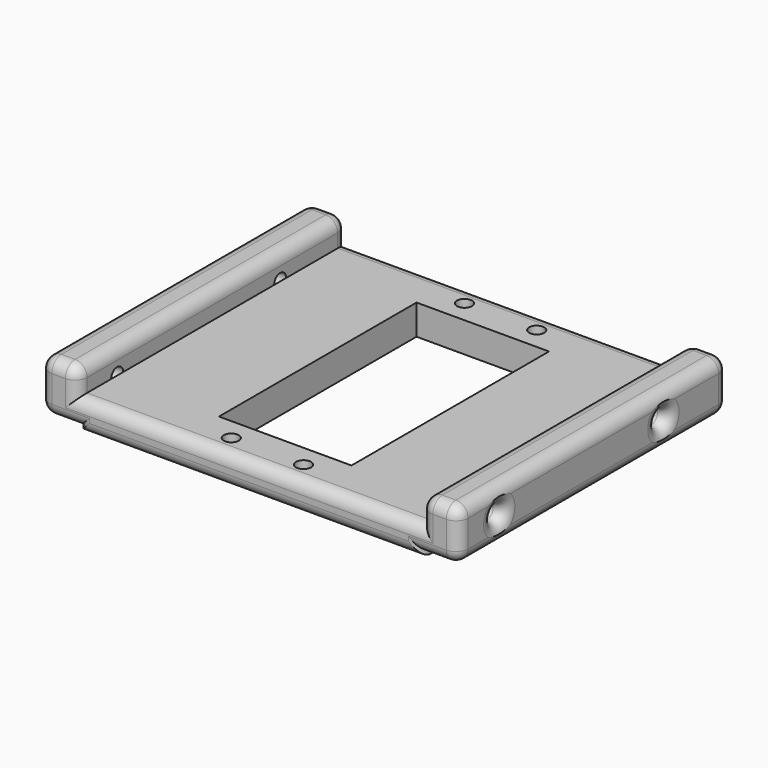
from build123d import *

# Parameters (mm, degrees)
F0_W           = 57
F0_H           = 56
F0_W_2         = 22
F0_H_2         = 41
F1_DEPTH       = 5
F3_W           = 56
F3_H           = 8.5
F4_DEPTH       = 6.25
F6_W           = 56
F6_H           = 8.5
F7_DEPTH       = 6.25
F8_D           = 2.5
F9_D           = 2.5
F9_DEPTH       = 6.251
F10_D          = 2.5
F10_DEPTH      = 6.251
F11_T1_DEPTH   = 2.25
F11_T3_DEPTH   = 52
F11_T5_DEPTH   = 4.5
F11_T7_DEPTH   = 5.75
F11_T9_DEPTH   = 67
F11_T11_DEPTH  = 4.25
F11_T13_DEPTH  = 2.25
F11_T15_DEPTH  = 57
F11_T17_DEPTH  = 2.25
F11_T19_DEPTH  = 4.25
F11_S23_W      = 2
F11_S23_H      = 2
F11_T24_DEPTH  = 2
F11_S29_W      = 2
F11_S29_H      = 2
F11_T30_DEPTH  = 2
F11_S35_W      = 2
F11_S35_H      = 2
F11_T36_DEPTH  = 2
F11_S41_W      = 2
F11_S41_H      = 2
F11_T42_DEPTH  = 2
F11_S47_W      = 2
F11_S47_H      = 2
F11_T48_DEPTH  = 2
F11_S53_W      = 2
F11_S53_H      = 2
F11_T54_DEPTH  = 2
F11_S59_W      = 2
F11_S59_H      = 2
F11_T60_DEPTH  = 2
F11_S65_W      = 2
F11_S65_H      = 2
F11_T66_DEPTH  = 2
F11_S71_W      = 2
F11_S71_H      = 2
F11_T72_DEPTH  = 2
F11_S77_W      = 2
F11_S77_H      = 2
F11_T78_DEPTH  = 2
F11_S83_W      = 2
F11_S83_H      = 2
F11_T84_DEPTH  = 2
F11_S89_W      = 2
F11_S89_H      = 2
F11_T90_DEPTH  = 2
F11_T105_DEPTH = 10.75
F11_T109_DEPTH = 9.25
F11_T116_DEPTH = 10.75
F11_T120_DEPTH = 9.25
F11_T127_DEPTH = 7.25
F11_T131_DEPTH = 62
F11_T138_DEPTH = 62
F11_T142_DEPTH = 7.25
F11_T149_DEPTH = 10.75
F11_T153_DEPTH = 9.25
F11_T160_DEPTH = 10.75
F11_T164_DEPTH = 9.25
F11_T171_DEPTH = 62
F11_T175_DEPTH = 7.25
F11_T182_DEPTH = 7.25
F11_T186_DEPTH = 62


# Not quite as in the source:
# - a fillet or chamfer that OpenCascade refuses, or shapes differently, is made with other operations: its cross-section is extruded or revolved along the edge and cut away or added


with BuildPart() as f1:
    # F0 (on Top) → F1 (new body)
    with BuildSketch(Plane.XY):
        Rectangle(F0_W, F0_H)
        Rectangle(F0_W_2, F0_H_2, mode=Mode.SUBTRACT)
    extrude(amount=-F1_DEPTH)

    # F3 (on offset) → F4 (join)
    with BuildSketch(Plane(origin=(-28.5, 0, 0), x_dir=(0, -1, 0), z_dir=(-1, 0, 0))):
        Rectangle(F3_W, F3_H)
    extrude(amount=F4_DEPTH)

    # F6 (on offset) → F7 (join)
    with BuildSketch(Plane.YZ.offset(28.5)):
        Rectangle(F6_W, F6_H)
    extrude(amount=F7_DEPTH)

    # F8 (through all)
    with Locations(Plane.XY):
        with Locations((6, 24.2), (-6, 24.2), (-6, -24.2), (6, -24.2)):
            Hole(F8_D / 2)

    # F9 (through all, one way)
    with BuildSketch(Plane(origin=(-28.5, 0, 0), x_dir=(0, -1, 0), z_dir=(1, 0, 0))):
        with Locations((-14.0771195292, 0), (19.7577979416, 0)):
            Circle(F9_D / 2)
    extrude(amount=-F9_DEPTH, mode=Mode.SUBTRACT)

    # F10 (through all, one way)
    with BuildSketch(Plane(origin=(28.5, 0, 0), x_dir=(0, 1, 0), z_dir=(-1, 0, 0))):
        with Locations((-19.5172671229, 0), (14.5558202639, 0)):
            Circle(F10_D / 2)
    extrude(amount=-F10_DEPTH, mode=Mode.SUBTRACT)

    # F11: fillet of radius 2 on 34 edges, made by hand

    # F11_s2 → F11_t1 (cut)
    with BuildSketch(Plane.YZ.offset(30.5)):
        with BuildLine():
            ThreePointArc((26, 4.25), (27.4142135624, 3.6642135624), (28, 2.25))
            Line((28, 2.25), (28, 4.25))
            Line((28, 4.25), (26, 4.25))
        make_face()
        with BuildLine():
            ThreePointArc((-28, 2.25), (-27.4142135624, 3.6642135624), (-26, 4.25))
            Line((-26, 4.25), (-28, 4.25))
            Line((-28, 4.25), (-28, 2.25))
        make_face()
    extrude(amount=F11_T1_DEPTH, mode=Mode.SUBTRACT)

    # F11_s4 → F11_t3 (cut)
    with BuildSketch(Plane.XZ.offset(-26)):
        with BuildLine():
            ThreePointArc((30.5, 4.25), (29.0857864376, 3.6642135624), (28.5, 2.25))
            Line((28.5, 2.25), (28.5, 4.25))
            Line((28.5, 4.25), (30.5, 4.25))
        make_face()
        with BuildLine():
            ThreePointArc((34.75, 2.25), (34.1642135624, 3.6642135624), (32.75, 4.25))
            Line((32.75, 4.25), (34.75, 4.25))
            Line((34.75, 4.25), (34.75, 2.25))
        make_face()
        with BuildLine():
            ThreePointArc((32.75, -4.25), (34.1642135624, -3.6642135624), (34.75, -2.25))
            Line((34.75, -2.25), (34.75, -4.25))
            Line((34.75, -4.25), (32.75, -4.25))
        make_face()
        with BuildLine():
            ThreePointArc((-28.5, 2.25), (-29.0857864376, 3.6642135624), (-30.5, 4.25))
            Line((-30.5, 4.25), (-28.5, 4.25))
            Line((-28.5, 4.25), (-28.5, 2.25))
        make_face()
        with BuildLine():
            ThreePointArc((-32.75, 4.25), (-34.1642135624, 3.6642135624), (-34.75, 2.25))
            Line((-34.75, 2.25), (-34.75, 4.25))
            Line((-34.75, 4.25), (-32.75, 4.25))
        make_face()
        with BuildLine():
            ThreePointArc((-34.75, -2.25), (-34.1642135624, -3.6642135624), (-32.75, -4.25))
            Line((-32.75, -4.25), (-34.75, -4.25))
            Line((-34.75, -4.25), (-34.75, -2.25))
        make_face()
    extrude(amount=F11_T3_DEPTH, mode=Mode.SUBTRACT)

    # F11_s6 → F11_t5 (cut)
    with BuildSketch(Plane.XY.offset(-2.25)):
        with BuildLine():
            ThreePointArc((32.75, -28), (34.1642135624, -27.4142135624), (34.75, -26))
            Line((34.75, -26), (34.75, -28))
            Line((34.75, -28), (32.75, -28))
        make_face()
        with BuildLine():
            ThreePointArc((34.75, 26), (34.1642135624, 27.4142135624), (32.75, 28))
            Line((32.75, 28), (34.75, 28))
            Line((34.75, 28), (34.75, 26))
        make_face()
        with BuildLine():
            ThreePointArc((-32.75, -28), (-34.1642135624, -27.4142135624), (-34.75, -26))
            Line((-34.75, -26), (-34.75, -28))
            Line((-34.75, -28), (-32.75, -28))
        make_face()
        with BuildLine():
            ThreePointArc((-34.75, 26), (-34.1642135624, 27.4142135624), (-32.75, 28))
            Line((-32.75, 28), (-34.75, 28))
            Line((-34.75, 28), (-34.75, 26))
        make_face()
    extrude(amount=F11_T5_DEPTH, mode=Mode.SUBTRACT)

    # F11_s8 → F11_t7 (cut)
    with BuildSketch(Plane.XY.offset(-10)):
        with BuildLine():
            ThreePointArc((-26.5, -28), (-27.9142135624, -27.4142135624), (-28.5, -26))
            Line((-28.5, -26), (-28.5, -28))
            Line((-28.5, -28), (-26.5, -28))
        make_face()
        with BuildLine():
            ThreePointArc((26.5, -28), (27.9142135624, -27.4142135624), (28.5, -26))
            Line((28.5, -26), (28.5, -28))
            Line((28.5, -28), (26.5, -28))
        make_face()
        with BuildLine():
            ThreePointArc((28.5, 26), (27.9142135624, 27.4142135624), (26.5, 28))
            Line((26.5, 28), (28.5, 28))
            Line((28.5, 28), (28.5, 26))
        make_face()
        with BuildLine():
            ThreePointArc((-28.5, 26), (-27.9142135624, 27.4142135624), (-26.5, 28))
            Line((-26.5, 28), (-28.5, 28))
            Line((-28.5, 28), (-28.5, 26))
        make_face()
    extrude(amount=F11_T7_DEPTH, mode=Mode.SUBTRACT)

    # F11_s10 → F11_t9 (cut)
    with BuildSketch(Plane.YZ.offset(-33.5)):
        with BuildLine():
            ThreePointArc((-28, -3), (-27.4142135624, -4.4142135624), (-26, -5))
            Line((-26, -5), (-28, -5))
            Line((-28, -5), (-28, -3))
        make_face()
        with BuildLine():
            ThreePointArc((26, -5), (27.4142135624, -4.4142135624), (28, -3))
            Line((28, -3), (28, -5))
            Line((28, -5), (26, -5))
        make_face()
    extrude(amount=F11_T9_DEPTH, mode=Mode.SUBTRACT)

    # F11_s12 → F11_t11 (cut)
    with BuildSketch(Plane.YZ.offset(28.5)):
        with BuildLine():
            ThreePointArc((-28, -2.25), (-27.4142135624, -3.6642135624), (-26, -4.25))
            Line((-26, -4.25), (-28, -4.25))
            Line((-28, -4.25), (-28, -2.25))
        make_face()
        with BuildLine():
            ThreePointArc((26, -4.25), (27.4142135624, -3.6642135624), (28, -2.25))
            Line((28, -2.25), (28, -4.25))
            Line((28, -4.25), (26, -4.25))
        make_face()
    extrude(amount=F11_T11_DEPTH, mode=Mode.SUBTRACT)

    # F11_s14 → F11_t13 (cut)
    with BuildSketch(Plane.XY):
        with BuildLine():
            ThreePointArc((30.5, -28), (29.0857864376, -27.4142135624), (28.5, -26))
            Line((28.5, -26), (28.5, -28))
            Line((28.5, -28), (30.5, -28))
        make_face()
        with BuildLine():
            ThreePointArc((-30.5, -28), (-29.0857864376, -27.4142135624), (-28.5, -26))
            Line((-28.5, -26), (-28.5, -28))
            Line((-28.5, -28), (-30.5, -28))
        make_face()
        with BuildLine():
            ThreePointArc((-28.5, 26), (-29.0857864376, 27.4142135624), (-30.5, 28))
            Line((-30.5, 28), (-28.5, 28))
            Line((-28.5, 28), (-28.5, 26))
        make_face()
        with BuildLine():
            ThreePointArc((28.5, 26), (29.0857864376, 27.4142135624), (30.5, 28))
            Line((30.5, 28), (28.5, 28))
            Line((28.5, 28), (28.5, 26))
        make_face()
    extrude(amount=F11_T13_DEPTH, mode=Mode.SUBTRACT)

    # F11_s16 → F11_t15 (cut)
    with BuildSketch(Plane.YZ.offset(-28.5)):
        with BuildLine():
            ThreePointArc((-28, -2), (-27.4142135624, -0.5857864376), (-26, 0))
            Line((-26, 0), (-28, 0))
            Line((-28, 0), (-28, -2))
        make_face()
        with BuildLine():
            ThreePointArc((26, 0), (27.4142135624, -0.5857864376), (28, -2))
            Line((28, -2), (28, 0))
            Line((28, 0), (26, 0))
        make_face()
    extrude(amount=F11_T15_DEPTH, mode=Mode.SUBTRACT)

    # F11_s18 → F11_t17 (cut)
    with BuildSketch(Plane.YZ.offset(-32.75)):
        with BuildLine():
            ThreePointArc((-28, 2.25), (-27.4142135624, 3.6642135624), (-26, 4.25))
            Line((-26, 4.25), (-28, 4.25))
            Line((-28, 4.25), (-28, 2.25))
        make_face()
        with BuildLine():
            ThreePointArc((26, 4.25), (27.4142135624, 3.6642135624), (28, 2.25))
            Line((28, 2.25), (28, 4.25))
            Line((28, 4.25), (26, 4.25))
        make_face()
    extrude(amount=F11_T17_DEPTH, mode=Mode.SUBTRACT)

    # F11_s20 → F11_t19 (cut)
    with BuildSketch(Plane.YZ.offset(-32.75)):
        with BuildLine():
            ThreePointArc((-28, -2.25), (-27.4142135624, -3.6642135624), (-26, -4.25))
            Line((-26, -4.25), (-28, -4.25))
            Line((-28, -4.25), (-28, -2.25))
        make_face()
        with BuildLine():
            ThreePointArc((26, -4.25), (27.4142135624, -3.6642135624), (28, -2.25))
            Line((28, -2.25), (28, -4.25))
            Line((28, -4.25), (26, -4.25))
        make_face()
    extrude(amount=F11_T19_DEPTH, mode=Mode.SUBTRACT)


with BuildPart() as f11_tool22:
    # F11_s23 → F11_t24 (new body)
    with BuildSketch(Plane.XZ.offset(-26)):
        with Locations((29.5, 3.25)):
            Rectangle(F11_S23_W, F11_S23_H)
    extrude(amount=-F11_T24_DEPTH)

    # F11_s25 → F11_t26 (revolve, cut)
    with BuildSketch(Plane(origin=(30.5, 26, 2.25), x_dir=(0.7071067812, 0, -0.7071067812), z_dir=(0.7071067812, 0, 0.7071067812))):
        with BuildLine():
            ThreePointArc((0, -2), (2, 0), (0, 2))
            Line((0, 2), (0, -2))
        make_face()
    revolve(axis=Axis((30.5, 26, 2.25), (0, 1, 0)), mode=Mode.SUBTRACT)


with BuildPart() as f1_1:
    add(f1.part)

    # F11_t21: cut F11_tool22
    add(f11_tool22.part, mode=Mode.SUBTRACT)


with BuildPart() as f11_tool28:
    # F11_s29 → F11_t30 (new body)
    with BuildSketch(Plane.YZ.offset(32.75)):
        with Locations((27, 3.25)):
            Rectangle(F11_S29_W, F11_S29_H)
    extrude(amount=F11_T30_DEPTH)

    # F11_s31 → F11_t32 (revolve, cut)
    with BuildSketch(Plane(origin=(32.75, 26, 2.25), x_dir=(0, -0.7071067812, -0.7071067812), z_dir=(0, -0.7071067812, 0.7071067812))):
        with BuildLine():
            ThreePointArc((0, -2), (2, 0), (0, 2))
            Line((0, 2), (0, -2))
        make_face()
    revolve(axis=Axis((32.75, 26, 2.25), (1, 0, 0)), mode=Mode.SUBTRACT)


with BuildPart() as f1_2:
    add(f1_1.part)

    # F11_t27: cut F11_tool28
    add(f11_tool28.part, mode=Mode.SUBTRACT)


with BuildPart() as f11_tool34:
    # F11_s35 → F11_t36 (new body)
    with BuildSketch(Plane.XZ.offset(26)):
        with Locations((29.5, 3.25)):
            Rectangle(F11_S35_W, F11_S35_H)
    extrude(amount=F11_T36_DEPTH)

    # F11_s37 → F11_t38 (revolve, cut)
    with BuildSketch(Plane(origin=(30.5, -26, 2.25), x_dir=(0.7071067812, 0, -0.7071067812), z_dir=(-0.7071067812, 0, -0.7071067812))):
        with BuildLine():
            ThreePointArc((0, -2), (2, 0), (0, 2))
            Line((0, 2), (0, -2))
        make_face()
    revolve(axis=Axis((30.5, -26, 2.25), (0, -1, 0)), mode=Mode.SUBTRACT)


with BuildPart() as f1_3:
    add(f1_2.part)

    # F11_t33: cut F11_tool34
    add(f11_tool34.part, mode=Mode.SUBTRACT)


with BuildPart() as f11_tool40:
    # F11_s41 → F11_t42 (new body)
    with BuildSketch(Plane.XZ.offset(26)):
        with Locations((33.75, 3.25)):
            Rectangle(F11_S41_W, F11_S41_H)
    extrude(amount=F11_T42_DEPTH)

    # F11_s43 → F11_t44 (revolve, cut)
    with BuildSketch(Plane(origin=(32.75, -26, 2.25), x_dir=(-0.7071067812, 0, -0.7071067812), z_dir=(-0.7071067812, 0, 0.7071067812))):
        with BuildLine():
            ThreePointArc((0, -2), (2, 0), (0, 2))
            Line((0, 2), (0, -2))
        make_face()
    revolve(axis=Axis((32.75, -26, 2.25), (0, -1, 0)), mode=Mode.SUBTRACT)


with BuildPart() as f1_4:
    add(f1_3.part)

    # F11_t39: cut F11_tool40
    add(f11_tool40.part, mode=Mode.SUBTRACT)


with BuildPart() as f11_tool46:
    # F11_s47 → F11_t48 (new body)
    with BuildSketch(Plane.XZ.offset(26)):
        with Locations((33.75, -3.25)):
            Rectangle(F11_S47_W, F11_S47_H)
    extrude(amount=F11_T48_DEPTH)

    # F11_s49 → F11_t50 (revolve, cut)
    with BuildSketch(Plane(origin=(32.75, -26, -2.25), x_dir=(-0.7071067812, 0, 0.7071067812), z_dir=(0.7071067812, 0, 0.7071067812))):
        with BuildLine():
            ThreePointArc((0, -2), (2, 0), (0, 2))
            Line((0, 2), (0, -2))
        make_face()
    revolve(axis=Axis((32.75, -26, -2.25), (0, -1, 0)), mode=Mode.SUBTRACT)


with BuildPart() as f1_5:
    add(f1_4.part)

    # F11_t45: cut F11_tool46
    add(f11_tool46.part, mode=Mode.SUBTRACT)


with BuildPart() as f11_tool52:
    # F11_s53 → F11_t54 (new body)
    with BuildSketch(Plane.XZ.offset(-26)):
        with Locations((33.75, -3.25)):
            Rectangle(F11_S53_W, F11_S53_H)
    extrude(amount=-F11_T54_DEPTH)

    # F11_s55 → F11_t56 (revolve, cut)
    with BuildSketch(Plane(origin=(32.75, 26, -2.25), x_dir=(-0.7071067812, 0, 0.7071067812), z_dir=(-0.7071067812, 0, -0.7071067812))):
        with BuildLine():
            ThreePointArc((0, -2), (2, 0), (0, 2))
            Line((0, 2), (0, -2))
        make_face()
    revolve(axis=Axis((32.75, 26, -2.25), (0, 1, 0)), mode=Mode.SUBTRACT)


with BuildPart() as f1_6:
    add(f1_5.part)

    # F11_t51: cut F11_tool52
    add(f11_tool52.part, mode=Mode.SUBTRACT)


with BuildPart() as f11_tool58:
    # F11_s59 → F11_t60 (new body)
    with BuildSketch(Plane.XZ.offset(26)):
        with Locations((-29.5, 3.25)):
            Rectangle(F11_S59_W, F11_S59_H)
    extrude(amount=F11_T60_DEPTH)

    # F11_s61 → F11_t62 (revolve, cut)
    with BuildSketch(Plane(origin=(-30.5, -26, 2.25), x_dir=(-0.7071067812, 0, -0.7071067812), z_dir=(-0.7071067812, 0, 0.7071067812))):
        with BuildLine():
            ThreePointArc((0, -2), (2, 0), (0, 2))
            Line((0, 2), (0, -2))
        make_face()
    revolve(axis=Axis((-30.5, -26, 2.25), (0, -1, 0)), mode=Mode.SUBTRACT)


with BuildPart() as f1_7:
    add(f1_6.part)

    # F11_t57: cut F11_tool58
    add(f11_tool58.part, mode=Mode.SUBTRACT)


with BuildPart() as f11_tool64:
    # F11_s65 → F11_t66 (new body)
    with BuildSketch(Plane.XZ.offset(26)):
        with Locations((-33.75, 3.25)):
            Rectangle(F11_S65_W, F11_S65_H)
    extrude(amount=F11_T66_DEPTH)

    # F11_s67 → F11_t68 (revolve, cut)
    with BuildSketch(Plane(origin=(-32.75, -26, 2.25), x_dir=(0.7071067812, 0, -0.7071067812), z_dir=(-0.7071067812, 0, -0.7071067812))):
        with BuildLine():
            ThreePointArc((0, -2), (2, 0), (0, 2))
            Line((0, 2), (0, -2))
        make_face()
    revolve(axis=Axis((-32.75, -26, 2.25), (0, -1, 0)), mode=Mode.SUBTRACT)


with BuildPart() as f1_8:
    add(f1_7.part)

    # F11_t63: cut F11_tool64
    add(f11_tool64.part, mode=Mode.SUBTRACT)


with BuildPart() as f11_tool70:
    # F11_s71 → F11_t72 (new body)
    with BuildSketch(Plane.XZ.offset(26)):
        with Locations((-33.75, -3.25)):
            Rectangle(F11_S71_W, F11_S71_H)
    extrude(amount=F11_T72_DEPTH)

    # F11_s73 → F11_t74 (revolve, cut)
    with BuildSketch(Plane(origin=(-32.75, -26, -2.25), x_dir=(0.7071067812, 0, 0.7071067812), z_dir=(0.7071067812, 0, -0.7071067812))):
        with BuildLine():
            ThreePointArc((0, -2), (2, 0), (0, 2))
            Line((0, 2), (0, -2))
        make_face()
    revolve(axis=Axis((-32.75, -26, -2.25), (0, -1, 0)), mode=Mode.SUBTRACT)


with BuildPart() as f1_9:
    add(f1_8.part)

    # F11_t69: cut F11_tool70
    add(f11_tool70.part, mode=Mode.SUBTRACT)


with BuildPart() as f11_tool76:
    # F11_s77 → F11_t78 (new body)
    with BuildSketch(Plane.YZ.offset(-32.75)):
        with Locations((27, -3.25)):
            Rectangle(F11_S77_W, F11_S77_H)
    extrude(amount=-F11_T78_DEPTH)

    # F11_s79 → F11_t80 (revolve, cut)
    with BuildSketch(Plane(origin=(-32.75, 26, -2.25), x_dir=(0, -0.7071067812, 0.7071067812), z_dir=(0, -0.7071067812, -0.7071067812))):
        with BuildLine():
            ThreePointArc((0, -2), (2, 0), (0, 2))
            Line((0, 2), (0, -2))
        make_face()
    revolve(axis=Axis((-32.75, 26, -2.25), (-1, 0, 0)), mode=Mode.SUBTRACT)


with BuildPart() as f1_10:
    add(f1_9.part)

    # F11_t75: cut F11_tool76
    add(f11_tool76.part, mode=Mode.SUBTRACT)


with BuildPart() as f11_tool82:
    # F11_s83 → F11_t84 (new body)
    with BuildSketch(Plane.XY.offset(2.25)):
        with Locations((-33.75, 27)):
            Rectangle(F11_S83_W, F11_S83_H)
    extrude(amount=F11_T84_DEPTH)

    # F11_s85 → F11_t86 (revolve, cut)
    with BuildSketch(Plane(origin=(-32.75, 26, 2.25), x_dir=(0.7071067812, -0.7071067812, 0), z_dir=(-0.7071067812, -0.7071067812, 0))):
        with BuildLine():
            ThreePointArc((0, -2), (2, 0), (0, 2))
            Line((0, 2), (0, -2))
        make_face()
    revolve(axis=Axis((-32.75, 26, 2.25), (0, 0, 1)), mode=Mode.SUBTRACT)


with BuildPart() as f1_11:
    add(f1_10.part)

    # F11_t81: cut F11_tool82
    add(f11_tool82.part, mode=Mode.SUBTRACT)


with BuildPart() as f11_tool88:
    # F11_s89 → F11_t90 (new body)
    with BuildSketch(Plane.YZ.offset(-30.5)):
        with Locations((27, 3.25)):
            Rectangle(F11_S89_W, F11_S89_H)
    extrude(amount=F11_T90_DEPTH)

    # F11_s91 → F11_t92 (revolve, cut)
    with BuildSketch(Plane(origin=(-30.5, 26, 2.25), x_dir=(0, -0.7071067812, -0.7071067812), z_dir=(0, -0.7071067812, 0.7071067812))):
        with BuildLine():
            ThreePointArc((0, -2), (2, 0), (0, 2))
            Line((0, 2), (0, -2))
        make_face()
    revolve(axis=Axis((-30.5, 26, 2.25), (1, 0, 0)), mode=Mode.SUBTRACT)


with BuildPart() as f1_12:
    add(f1_11.part)

    # F11_t87: cut F11_tool88
    add(f11_tool88.part, mode=Mode.SUBTRACT)

    # F11_s93 → F11_t94 (revolve, cut)
    with BuildSketch(Plane.XY):
        with BuildLine():
            ThreePointArc((34.75, -16.2672671229), (34.1642135624, -17.6814806852), (32.75, -18.2672671229))
            Line((32.75, -18.2672671229), (34.75, -18.2672671229))
            Line((34.75, -18.2672671229), (34.75, -16.2672671229))
        make_face()
    revolve(axis=Axis((34.75, -19.5172671229, 0), (-1, 0, 0)), mode=Mode.SUBTRACT)

    # F11_s95 → F11_t96 (revolve, cut)
    with BuildSketch(Plane.XY):
        with BuildLine():
            ThreePointArc((34.75, 17.8058202639), (34.1642135624, 16.3916067015), (32.75, 15.8058202639))
            Line((32.75, 15.8058202639), (34.75, 15.8058202639))
            Line((34.75, 15.8058202639), (34.75, 17.8058202639))
        make_face()
    revolve(axis=Axis((34.75, 14.5558202639, 0), (-1, 0, 0)), mode=Mode.SUBTRACT)

    # F11_s97 → F11_t98 (revolve, cut)
    with BuildSketch(Plane.XY):
        with BuildLine():
            ThreePointArc((-34.75, 10.8271195292), (-34.1642135624, 12.2413330916), (-32.75, 12.8271195292))
            Line((-32.75, 12.8271195292), (-34.75, 12.8271195292))
            Line((-34.75, 12.8271195292), (-34.75, 10.8271195292))
        make_face()
    revolve(axis=Axis((-34.75, 14.0771195292, 0), (1, 0, 0)), mode=Mode.SUBTRACT)

    # F11_s99 → F11_t100 (revolve, cut)
    with BuildSketch(Plane.XY):
        with BuildLine():
            ThreePointArc((-34.75, -23.0077979416), (-34.1642135624, -21.5935843792), (-32.75, -21.0077979416))
            Line((-32.75, -21.0077979416), (-34.75, -21.0077979416))
            Line((-34.75, -21.0077979416), (-34.75, -23.0077979416))
        make_face()
    revolve(axis=Axis((-34.75, -19.7577979416, 0), (1, 0, 0)), mode=Mode.SUBTRACT)


with BuildPart() as f11_tool103:
    # F11_s104 → F11_t105 (new body)
    with BuildSketch(Plane.XY.offset(0.75)):
        with BuildLine():
            ThreePointArc((-26.5, -28), (-27.9142135624, -27.4142135624), (-28.5, -26))
            Line((-28.5, -26), (-28.5, -28))
            Line((-28.5, -28), (-26.5, -28))
        make_face()
    extrude(amount=-F11_T105_DEPTH)

    split(bisect_by=Plane.XY.offset(-4.25), keep=Keep.TOP)


with BuildPart() as f11_tool107:
    # F11_s108 → F11_t109 (new body)
    with BuildSketch(Plane.YZ.offset(-23.5)):
        with BuildLine():
            ThreePointArc((-28, -2.25), (-27.4142135624, -3.6642135624), (-26, -4.25))
            Line((-26, -4.25), (-28, -4.25))
            Line((-28, -4.25), (-28, -2.25))
        make_face()
    extrude(amount=-F11_T109_DEPTH)

    split(bisect_by=Plane.YZ.offset(-28.5), keep=Keep.TOP)


with BuildPart() as f11_tool103_1:
    add(f11_tool103.part)

    # F11_t111: intersect F11_tool107
    add(f11_tool107.part, mode=Mode.INTERSECT)


with BuildPart() as f1_13:
    add(f1_12.part)

    # F11_t101: cut F11_tool103
    add(f11_tool103_1.part, mode=Mode.SUBTRACT)


with BuildPart() as f11_tool114:
    # F11_s115 → F11_t116 (new body)
    with BuildSketch(Plane.XY.offset(0.75)):
        with BuildLine():
            ThreePointArc((26.5, -28), (27.9142135624, -27.4142135624), (28.5, -26))
            Line((28.5, -26), (28.5, -28))
            Line((28.5, -28), (26.5, -28))
        make_face()
    extrude(amount=-F11_T116_DEPTH)

    split(bisect_by=Plane.XY.offset(-4.25), keep=Keep.TOP)


with BuildPart() as f11_tool118:
    # F11_s119 → F11_t120 (new body)
    with BuildSketch(Plane.YZ.offset(23.5)):
        with BuildLine():
            ThreePointArc((-28, -2.25), (-27.4142135624, -3.6642135624), (-26, -4.25))
            Line((-26, -4.25), (-28, -4.25))
            Line((-28, -4.25), (-28, -2.25))
        make_face()
    extrude(amount=F11_T120_DEPTH)

    split(bisect_by=Plane.YZ.offset(28.5), keep=Keep.BOTTOM)


with BuildPart() as f11_tool114_1:
    add(f11_tool114.part)

    # F11_t122: intersect F11_tool118
    add(f11_tool118.part, mode=Mode.INTERSECT)


with BuildPart() as f1_14:
    add(f1_13.part)

    # F11_t112: cut F11_tool114
    add(f11_tool114_1.part, mode=Mode.SUBTRACT)


with BuildPart() as f11_tool125:
    # F11_s126 → F11_t127 (new body)
    with BuildSketch(Plane.XY.offset(2.25)):
        with BuildLine():
            ThreePointArc((30.5, -28), (29.0857864376, -27.4142135624), (28.5, -26))
            Line((28.5, -26), (28.5, -28))
            Line((28.5, -28), (30.5, -28))
        make_face()
    extrude(amount=-F11_T127_DEPTH)

    split(bisect_by=Plane.XY, keep=Keep.BOTTOM)


with BuildPart() as f11_tool129:
    # F11_s130 → F11_t131 (new body)
    with BuildSketch(Plane.YZ.offset(-28.5)):
        with BuildLine():
            ThreePointArc((-28, -2), (-27.4142135624, -0.5857864376), (-26, 0))
            Line((-26, 0), (-28, 0))
            Line((-28, 0), (-28, -2))
        make_face()
    extrude(amount=F11_T131_DEPTH)

    split(bisect_by=Plane.YZ.offset(28.5), keep=Keep.TOP)


with BuildPart() as f11_tool125_1:
    add(f11_tool125.part)

    # F11_t133: intersect F11_tool129
    add(f11_tool129.part, mode=Mode.INTERSECT)


with BuildPart() as f1_15:
    add(f1_14.part)

    # F11_t123: cut F11_tool125
    add(f11_tool125_1.part, mode=Mode.SUBTRACT)


with BuildPart() as f11_tool136:
    # F11_s137 → F11_t138 (new body)
    with BuildSketch(Plane.YZ.offset(-33.5)):
        with BuildLine():
            ThreePointArc((-28, -2), (-27.4142135624, -0.5857864376), (-26, 0))
            Line((-26, 0), (-28, 0))
            Line((-28, 0), (-28, -2))
        make_face()
    extrude(amount=F11_T138_DEPTH)

    split(bisect_by=Plane.YZ.offset(-28.5), keep=Keep.BOTTOM)


with BuildPart() as f11_tool140:
    # F11_s141 → F11_t142 (new body)
    with BuildSketch(Plane.XY.offset(-5)):
        with BuildLine():
            ThreePointArc((-30.5, -28), (-29.0857864376, -27.4142135624), (-28.5, -26))
            Line((-28.5, -26), (-28.5, -28))
            Line((-28.5, -28), (-30.5, -28))
        make_face()
    extrude(amount=F11_T142_DEPTH)

    split(bisect_by=Plane.XY, keep=Keep.BOTTOM)


with BuildPart() as f11_tool136_1:
    add(f11_tool136.part)

    # F11_t144: intersect F11_tool140
    add(f11_tool140.part, mode=Mode.INTERSECT)


with BuildPart() as f1_16:
    add(f1_15.part)

    # F11_t134: cut F11_tool136
    add(f11_tool136_1.part, mode=Mode.SUBTRACT)


with BuildPart() as f11_tool147:
    # F11_s148 → F11_t149 (new body)
    with BuildSketch(Plane.XY.offset(0.75)):
        with BuildLine():
            ThreePointArc((28.5, 26), (27.9142135624, 27.4142135624), (26.5, 28))
            Line((26.5, 28), (28.5, 28))
            Line((28.5, 28), (28.5, 26))
        make_face()
    extrude(amount=-F11_T149_DEPTH)

    split(bisect_by=Plane.XY.offset(-4.25), keep=Keep.TOP)


with BuildPart() as f11_tool151:
    # F11_s152 → F11_t153 (new body)
    with BuildSketch(Plane.YZ.offset(23.5)):
        with BuildLine():
            ThreePointArc((26, -4.25), (27.4142135624, -3.6642135624), (28, -2.25))
            Line((28, -2.25), (28, -4.25))
            Line((28, -4.25), (26, -4.25))
        make_face()
    extrude(amount=F11_T153_DEPTH)

    split(bisect_by=Plane.YZ.offset(28.5), keep=Keep.BOTTOM)


with BuildPart() as f11_tool147_1:
    add(f11_tool147.part)

    # F11_t155: intersect F11_tool151
    add(f11_tool151.part, mode=Mode.INTERSECT)


with BuildPart() as f1_17:
    add(f1_16.part)

    # F11_t145: cut F11_tool147
    add(f11_tool147_1.part, mode=Mode.SUBTRACT)


with BuildPart() as f11_tool158:
    # F11_s159 → F11_t160 (new body)
    with BuildSketch(Plane.XY.offset(0.75)):
        with BuildLine():
            ThreePointArc((-28.5, 26), (-27.9142135624, 27.4142135624), (-26.5, 28))
            Line((-26.5, 28), (-28.5, 28))
            Line((-28.5, 28), (-28.5, 26))
        make_face()
    extrude(amount=-F11_T160_DEPTH)

    split(bisect_by=Plane.XY.offset(-4.25), keep=Keep.TOP)


with BuildPart() as f11_tool162:
    # F11_s163 → F11_t164 (new body)
    with BuildSketch(Plane.YZ.offset(-23.5)):
        with BuildLine():
            ThreePointArc((26, -4.25), (27.4142135624, -3.6642135624), (28, -2.25))
            Line((28, -2.25), (28, -4.25))
            Line((28, -4.25), (26, -4.25))
        make_face()
    extrude(amount=-F11_T164_DEPTH)

    split(bisect_by=Plane.YZ.offset(-28.5), keep=Keep.TOP)


with BuildPart() as f11_tool158_1:
    add(f11_tool158.part)

    # F11_t166: intersect F11_tool162
    add(f11_tool162.part, mode=Mode.INTERSECT)


with BuildPart() as f1_18:
    add(f1_17.part)

    # F11_t156: cut F11_tool158
    add(f11_tool158_1.part, mode=Mode.SUBTRACT)


with BuildPart() as f11_tool169:
    # F11_s170 → F11_t171 (new body)
    with BuildSketch(Plane.YZ.offset(28.5)):
        with BuildLine():
            ThreePointArc((26, 0), (27.4142135624, -0.5857864376), (28, -2))
            Line((28, -2), (28, 0))
            Line((28, 0), (26, 0))
        make_face()
    extrude(amount=-F11_T171_DEPTH)

    split(bisect_by=Plane.YZ.offset(-28.5), keep=Keep.BOTTOM)


with BuildPart() as f11_tool173:
    # F11_s174 → F11_t175 (new body)
    with BuildSketch(Plane.XY.offset(2.25)):
        with BuildLine():
            ThreePointArc((-28.5, 26), (-29.0857864376, 27.4142135624), (-30.5, 28))
            Line((-30.5, 28), (-28.5, 28))
            Line((-28.5, 28), (-28.5, 26))
        make_face()
    extrude(amount=-F11_T175_DEPTH)

    split(bisect_by=Plane.XY, keep=Keep.BOTTOM)


with BuildPart() as f11_tool169_1:
    add(f11_tool169.part)

    # F11_t177: intersect F11_tool173
    add(f11_tool173.part, mode=Mode.INTERSECT)


with BuildPart() as f1_19:
    add(f1_18.part)

    # F11_t167: cut F11_tool169
    add(f11_tool169_1.part, mode=Mode.SUBTRACT)


with BuildPart() as f11_tool180:
    # F11_s181 → F11_t182 (new body)
    with BuildSketch(Plane.XY.offset(-5)):
        with BuildLine():
            ThreePointArc((28.5, 26), (29.0857864376, 27.4142135624), (30.5, 28))
            Line((30.5, 28), (28.5, 28))
            Line((28.5, 28), (28.5, 26))
        make_face()
    extrude(amount=F11_T182_DEPTH)

    split(bisect_by=Plane.XY, keep=Keep.BOTTOM)


with BuildPart() as f11_tool184:
    # F11_s185 → F11_t186 (new body)
    with BuildSketch(Plane.YZ.offset(33.5)):
        with BuildLine():
            ThreePointArc((26, 0), (27.4142135624, -0.5857864376), (28, -2))
            Line((28, -2), (28, 0))
            Line((28, 0), (26, 0))
        make_face()
    extrude(amount=-F11_T186_DEPTH)

    split(bisect_by=Plane.YZ.offset(28.5), keep=Keep.TOP)


with BuildPart() as f11_tool180_1:
    add(f11_tool180.part)

    # F11_t188: intersect F11_tool184
    add(f11_tool184.part, mode=Mode.INTERSECT)


with BuildPart() as f1_20:
    add(f1_19.part)

    # F11_t178: cut F11_tool180
    add(f11_tool180_1.part, mode=Mode.SUBTRACT)


solid = f1_20.part
